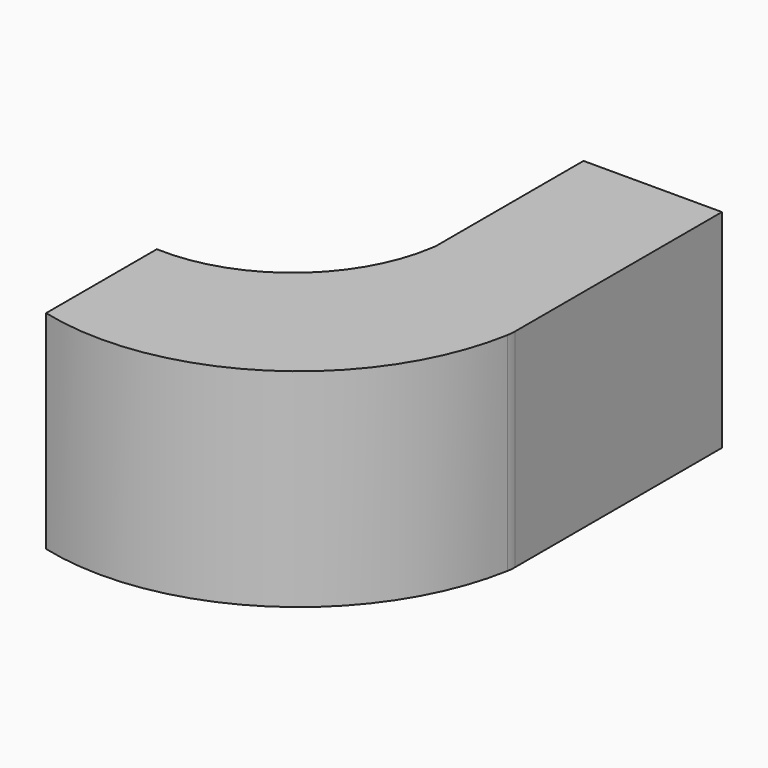
from build123d import *

# Parameters (mm, degrees)
F1_DEPTH = 9.525
F2_DEPTH = 57.15


# Not quite as in the source:
# - ends of sketch curves that miss each other by under 0.0002 mm in the source are joined


with BuildPart() as f1:
    # F0 (on Top) → F1 (new body)
    with BuildSketch(Plane.XY):
        with BuildLine():
            Line((-9.525, -40.8894196153), (-9.525, 101.6))
            Line((-9.525, 101.6), (-76.2, 101.6))
            Line((-76.2, 101.6), (-76.2, 1.7757813176))
            ThreePointArc((-76.2, 1.7757813176), (-76.2737613091, -0.1585489984), (-76.4946168324, -2.0816447683))
            ThreePointArc((-76.4946168324, -2.0816447683), (-107.8980822653, -57.1580249287), (-168.0578880185, -77.1675992495))
            Line((-168.0578880185, -77.1675992495), (-168.0578880185, -143.8425992495))
            ThreePointArc((-168.0578880185, -143.8425992495), (-66.0749732172, -127.3460628222), (-9.525, -40.8894196153))
        make_face()
    extrude(amount=F1_DEPTH)

    # F0 (on Top) → F2 (join)
    with BuildSketch(Plane.XY):
        with BuildLine():
            ThreePointArc((-2.87076e-05, -40.8894195721), (-7.1769e-06, -40.8703254289), (0, -40.8512312749))
            Line((0, -40.8512312749), (0, 101.6))
            Line((0, 101.6), (-9.525, 101.6))
            Line((-9.525, 101.6), (-9.525, -40.8894196153))
            Line((-9.525, -40.8894196153), (-2.87076e-05, -40.8894195721))
        make_face()
        with BuildLine():
            ThreePointArc((-0.3915773599, -45.2940678749), (-0.0997672663, -43.1002807673), (-2.87076e-05, -40.8894195721))
            Line((-2.87076e-05, -40.8894195721), (-9.525, -40.8894196153))
            ThreePointArc((-9.525, -40.8894196153), (-66.0749732172, -127.3460628222), (-168.0578880185, -143.8425992495))
            Line((-168.0578880185, -143.8425992495), (-168.0578880185, -153.3675992495))
            ThreePointArc((-168.0578880185, -153.3675992495), (-60.6607327041, -135.8882486075), (-0.3915773599, -45.2940678749))
        make_face()
    extrude(amount=F2_DEPTH)

    # F3: F1 across face


with BuildPart() as f1_1:
    add(f1.part)
    add(f1.part.mirror(Plane(origin=(-44.7738585302, -61.3523725629, 57.15), x_dir=(1, 0, 0), z_dir=(0, 0, 1))))


solid = f1_1.part
